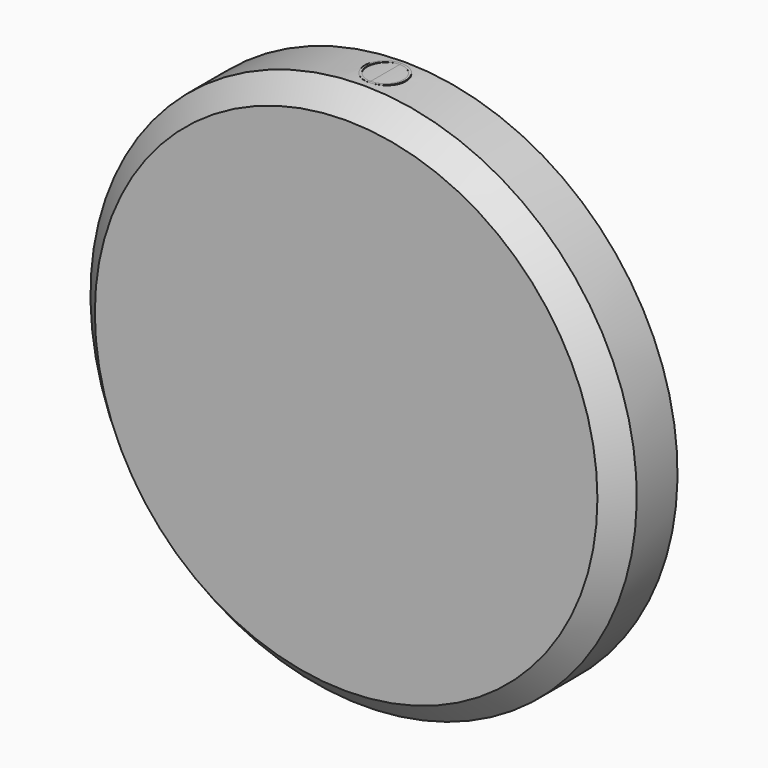
from build123d import *
from build123d import SkipClean  # not in build123d's __all__

# Parameters (mm, degrees)
F1_DEPTH = 10
F2_SIZE  = 3
F3_R     = 2.821
F3_R_2   = 2.5
F4_DEPTH = 37.5
F5_DEPTH = 75


with BuildPart() as f1:
    # F0 (on Front) → F1 (new body)
    with BuildSketch(Plane.XZ):
        with BuildLine():
            ThreePointArc((37.5, 0), (26.5165042945, 26.5165042945), (0, 37.5))
            Line((0, 37.5), (0, -37.5))
            ThreePointArc((0, -37.5), (26.5165042945, -26.5165042945), (37.5, 0))
        make_face()
        with BuildLine():
            Line((0, -37.5), (0, 37.5))
            ThreePointArc((0, 37.5), (-37.5, 0), (0, -37.5))
        make_face()
    extrude(amount=F1_DEPTH)

    # F2
    f2_edges = [f1.edges().sort_by_distance(p)[0] for p in [
        (-37.5, -10, 0),
    ]]
    chamfer(f2_edges, length=F2_SIZE)

    # F3 (on Top) → F4 (join, symmetric)
    with BuildSketch(Plane.XY):
        with Locations((0, -3.2904869877)):
            Circle(F3_R)
        with Locations((0, -3.2904869877)):
            Circle(F3_R_2, mode=Mode.SUBTRACT)
    with SkipClean():  # cleaning this boolean's faces spoils the solid; the shape is the same uncleaned
        extrude(amount=F4_DEPTH, both=True)

    # F5 (add): a face of the model
    f5_faces = [f1.faces().sort_by_distance(p)[0] for p in [
        (-0.0630794776, -0.6299869877, -37.5),
    ]]
    with SkipClean():  # cleaning this boolean's faces spoils the solid; the shape is the same uncleaned
        extrude(f5_faces, amount=-F5_DEPTH)


solid = f1.part
